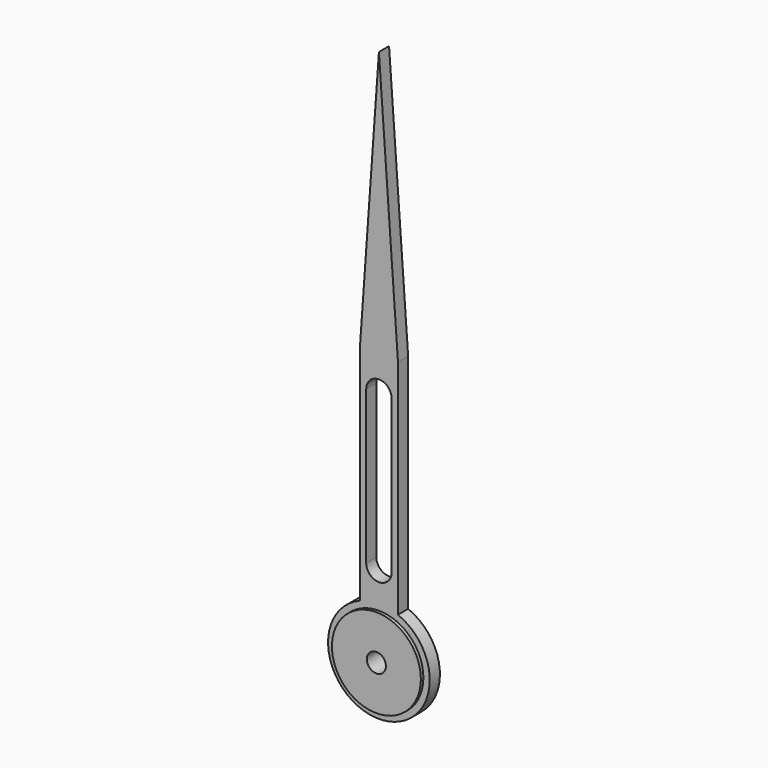
from build123d import *

# Parameters (mm, degrees)
F0_R     = 7
F0_R_2   = 1.5
F1_DEPTH = 1.5
F2_DEPTH = 1


# Not quite as in the source:
# - a feature names something its author has since deleted; it is built from what else it names


with BuildPart() as f1:
    # F0 (on Front) → F1 (new body, symmetric)
    with BuildSketch(Plane.XZ):
        with Locations((-19.8327995853, -33.1064267996)):
            Circle(F0_R)
        with Locations((-19.8327995853, -33.1064267996)):
            Circle(F0_R_2, mode=Mode.SUBTRACT)
    extrude(amount=F1_DEPTH, both=True)

    # F0 (on Front) → F2 (join, symmetric)
    with BuildSketch(Plane.XZ):
        with BuildLine():
            ThreePointArc((-22.8327995853, -25.6902283125), (-19.8327995853, -41.1064267996), (-16.8327995853, -25.6902283125))
            Line((-16.8327995853, -25.6902283125), (-16.8327995853, 9.3097716875))
            Line((-16.8327995853, 9.3097716875), (-19.8327995853, 51.3097716875))
            Line((-19.8327995853, 51.3097716875), (-22.8327995853, 9.3097716875))
            Line((-22.8327995853, 9.3097716875), (-22.8327995853, -25.6902283125))
        make_face()
        with Locations((-19.8327995853, -33.1064267996)):
            Circle(F0_R, mode=Mode.SUBTRACT)
        with BuildLine():
            ThreePointArc((-21.8327995853, 3.9472361095), (-19.8327995853, 5.9472361095), (-17.8327995853, 3.9472361095))
            Line((-17.8327995853, 3.9472361095), (-17.8327995853, -20.1542899013))
            ThreePointArc((-17.8327995853, -20.1542899013), (-19.8327995853, -22.1542899013), (-21.8327995853, -20.1542899013))
            Line((-21.8327995853, -20.1542899013), (-21.8327995853, 3.9472361095))
        make_face(mode=Mode.SUBTRACT)
    extrude(amount=F2_DEPTH, both=True)


solid = f1.part
